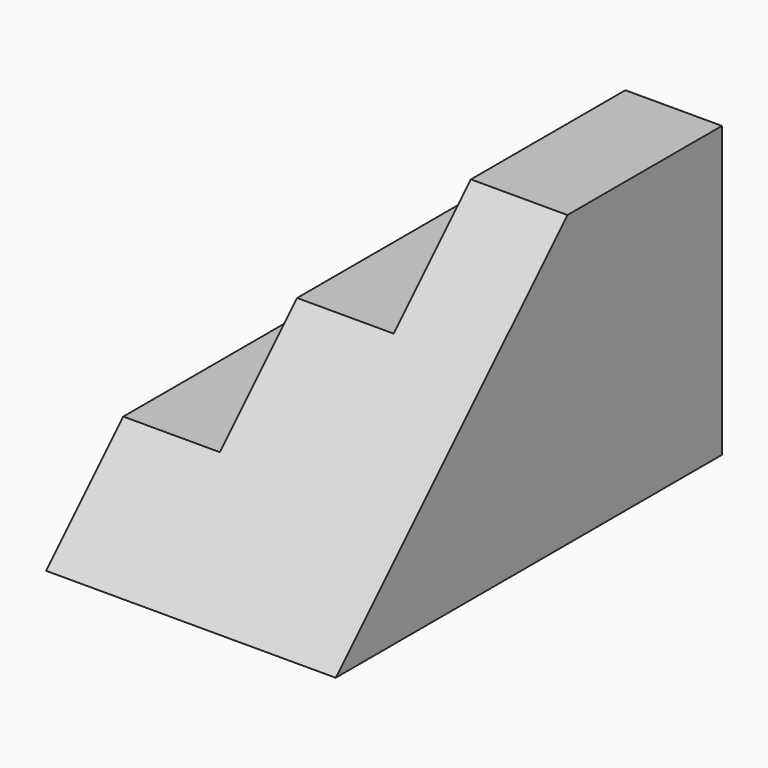
from build123d import *

# Parameters (mm, degrees)
F1_DEPTH = 100
F2_SIZE  = 59.99999


# Not quite as in the source:
# - a fillet or chamfer is up to 0.001 mm smaller than in the source, because OpenCascade refuses the exact size


with BuildPart() as f1:
    # F0 (on Front) → F1 (new body)
    with BuildSketch(Plane.XZ):
        Polygon((-60, 0), (0, 0), (0, 60), (-20, 60), (-20, 40), (-40, 40), (-40, 20), (-60, 20), align=None)
    extrude(amount=F1_DEPTH)

    # F2 (size 60 in the source; OpenCascade refuses exactly that, so slightly less here)
    f2_edges = [f1.edges().sort_by_distance(p)[0] for p in [
        (-10, -100, 60),
    ]]
    chamfer(f2_edges, length=F2_SIZE)


solid = f1.part
